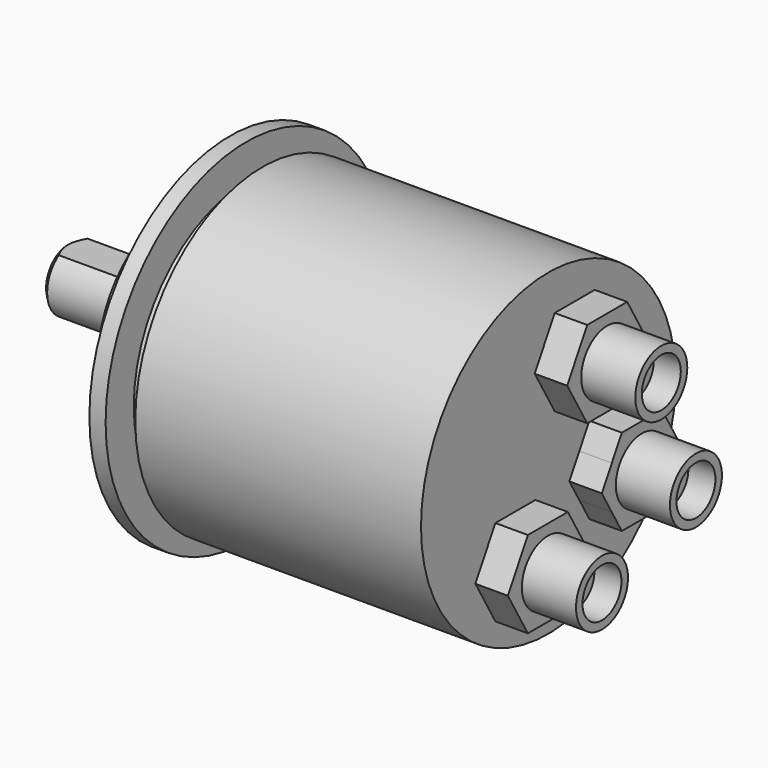
from build123d import *

# Parameters (mm, degrees)
F0_R        = 6
F1_DEPTH    = 18.9
F2_W        = 21.1690347642
F2_H        = 4.931249544
F3_DEPTH    = 18.901
F4_T2_ANGLE = 359.64
F5_R        = 7
F6_DEPTH    = 1.1
F7_R        = 18
F8_DEPTH    = 10
F9_R        = 32.5
F10_DEPTH   = 3
F11_R       = 26
F12_DEPTH   = 3
F14_R       = 29.4
F15_DEPTH   = 52.8
F16_R       = 1.75
F17_DEPTH   = 3
F19_DEPTH   = 6
F20_R       = 6
F21_DEPTH   = 10
F22_R       = 4.5
F23_DEPTH   = 5


# Not quite as in the source:
# - a fillet or chamfer that OpenCascade refuses, or shapes differently, is made with other operations: its cross-section is extruded or revolved along the edge and cut away or added


with BuildPart() as f1:
    # F0 (on Right) → F1 (new body)
    with BuildSketch(Plane.YZ):
        Circle(F0_R)
    extrude(amount=-F1_DEPTH)

    # F2 (on Right) → F3 (cut, through all)
    with BuildSketch(Plane.YZ):
        with Locations((0.0764410943, 7.465624772)):
            Rectangle(F2_W, F2_H)
    extrude(amount=-F3_DEPTH, mode=Mode.SUBTRACT)

    # F4: chamfer of 1 on 1 edges, made by hand

    # F4_s1 → F4_t2 (revolve, cut)
    with BuildSketch(Plane(origin=(0, 0, 0), x_dir=(1, 0, 0), z_dir=(0, 0.9999950652, 0.0031415875))):
        with BuildLine():
            Line((-17.8717157288, -6.0282842712), (-18.9282842712, -4.9717157288))
            Line((-18.9282842712, -4.9717157288), (-18.9482842712, -4.9717157288))
            ThreePointArc((-18.9482842712, -4.9717157288), (-18.92, -5.4858578644), (-18.92, -6))
            Line((-18.92, -6), (-18.9, -6.02))
            ThreePointArc((-18.9, -6.02), (-18.3858578644, -6.02), (-17.8717157288, -6.0482842712))
            Line((-17.8717157288, -6.0482842712), (-17.8717157288, -6.0282842712))
        make_face()
    revolve(axis=Axis((-18.9, 0, 0), (1, 0, 0)), revolution_arc=F4_T2_ANGLE, mode=Mode.SUBTRACT)

    # F5 (on face) → F6 (join)
    with BuildSketch(Plane.YZ):
        Circle(F5_R)
    extrude(amount=F6_DEPTH)

    # F7 (on face) → F8 (join)
    with BuildSketch(Plane.YZ.offset(1.1)):
        Circle(F7_R)
    extrude(amount=F8_DEPTH)

    # F9 (on face) → F10 (join)
    with BuildSketch(Plane.YZ.offset(11.1)):
        Circle(F9_R)
    extrude(amount=F10_DEPTH)

    # F11 (on face) → F12 (join)
    with BuildSketch(Plane.YZ.offset(14.1)):
        Circle(F11_R)
    extrude(amount=F12_DEPTH)

    # F14 (on offset) → F15 (join, through all)
    with BuildSketch(Plane(origin=(69.9, 0, 0), x_dir=(0, -1, 0), z_dir=(-1, 0, 0))):
        Circle(F14_R)
    extrude(amount=F15_DEPTH)

    # F16 (on face) → F17 (cut)
    with BuildSketch(Plane(origin=(11.1, 0, 0), x_dir=(0, -1, 0), z_dir=(-1, 0, 0))):
        with Locations((-24, 0)):
            Circle(F16_R)
        with Locations((12, -20.7846096908)):
            Circle(F16_R)
        with Locations((12, 20.7846096908)):
            Circle(F16_R)
    extrude(amount=-F17_DEPTH, mode=Mode.SUBTRACT)

    # F18 (on face) → F19 (join)
    with BuildSketch(Plane.YZ.offset(69.9)):
        with BuildLine():
            ThreePointArc((21.0282031968, -10.574938038), (21.8274066017, -8.6454903731), (22.1, -6.57493798))
            ThreePointArc((22.1, -6.57493798), (21.8274066078, -4.5043856099), (21.0282032207, -2.5749379634))
            ThreePointArc((21.0282032207, -2.5749379634), (18.0999999917, 0.3532652551), (14.1, 1.42506202))
            ThreePointArc((14.1, 1.42506202), (10.1000001451, 0.3532653341), (7.1717969373, -2.5749376897))
            ThreePointArc((7.1717969373, -2.5749376897), (6.1, -6.5749379695), (7.1717969269, -10.5749382522))
            ThreePointArc((7.1717969269, -10.5749382522), (10.1000001361, -13.5031412888), (14.1, -14.57493798))
            ThreePointArc((14.1, -14.57493798), (18.099999971, -13.503141227), (21.0282031968, -10.574938038))
        make_face()
        with BuildLine():
            ThreePointArc((21.0282032207, -2.5749379634), (21.8274066078, -4.5043856099), (22.1, -6.57493798))
            ThreePointArc((22.1, -6.57493798), (21.8274066017, -8.6454903731), (21.0282031968, -10.574938038))
            Line((21.0282031968, -10.574938038), (23.337604307, -6.57493798))
            Line((23.337604307, -6.57493798), (21.0282032207, -2.5749379634))
        make_face()
        with BuildLine():
            ThreePointArc((14.1, 1.42506202), (18.0999999917, 0.3532652551), (21.0282032207, -2.5749379634))
            Line((21.0282032207, -2.5749379634), (18.7188021535, 1.42506202))
            Line((18.7188021535, 1.42506202), (14.1, 1.42506202))
        make_face()
        with BuildLine():
            Line((18.7188021535, -14.57493798), (21.0282031968, -10.574938038))
            ThreePointArc((21.0282031968, -10.574938038), (18.099999971, -13.503141227), (14.1, -14.57493798))
            Line((14.1, -14.57493798), (18.7188021535, -14.57493798))
        make_face()
        with BuildLine():
            ThreePointArc((7.1717969373, -2.5749376897), (10.1000001451, 0.3532653341), (14.1, 1.42506202))
            Line((14.1, 1.42506202), (9.4811978465, 1.42506202))
            Line((9.4811978465, 1.42506202), (7.1717969373, -2.5749376897))
        make_face()
        with BuildLine():
            Line((9.4811978465, -14.57493798), (14.1, -14.57493798))
            ThreePointArc((14.1, -14.57493798), (10.1000001361, -13.5031412888), (7.1717969269, -10.5749382522))
            Line((7.1717969269, -10.5749382522), (9.4811978465, -14.57493798))
        make_face()
        with BuildLine():
            ThreePointArc((7.1717969269, -10.5749382522), (6.1, -6.5749379695), (7.1717969373, -2.5749376897))
            Line((7.1717969373, -2.5749376897), (4.862395693, -6.57493798))
            Line((4.862395693, -6.57493798), (7.1717969269, -10.5749382522))
        make_face()
        Polygon((10.7188021535, 22.2), (1.4811978465, 22.2), (-3.137604307, 14.2), (1.4811978465, 6.2), (10.7188021535, 6.2), (15.337604307, 14.2), align=None)
        Polygon((-2.9811978465, -6.4), (-12.2188021535, -6.4), (-16.837604307, -14.4), (-12.2188021535, -22.4), (-2.9811978465, -22.4), (1.637604307, -14.4), align=None)
    extrude(amount=F19_DEPTH)

    # F20 (on face) → F21 (join)
    with BuildSketch(Plane.YZ.offset(75.9)):
        with Locations((6.1, 14.2)):
            Circle(F20_R)
        with Locations((14.1, -6.57493798)):
            Circle(F20_R)
        with Locations((-7.6, -14.4)):
            Circle(F20_R)
    extrude(amount=F21_DEPTH)

    # F22 (on face) → F23 (cut)
    with BuildSketch(Plane.YZ.offset(85.9)):
        with Locations((6.1, 14.2)):
            Circle(F22_R)
        with Locations((-7.6, -14.4)):
            Circle(F22_R)
        with Locations((14.1, -6.57493798)):
            Circle(F22_R)
    extrude(amount=-F23_DEPTH, mode=Mode.SUBTRACT)


solid = f1.part
